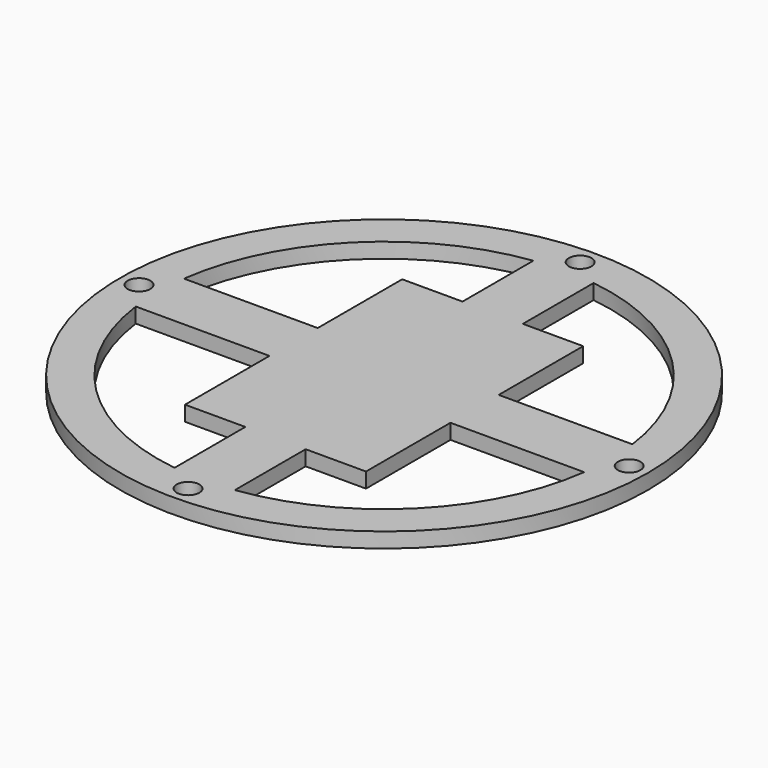
from build123d import *

# Parameters (mm, degrees)
F0_R     = 35
F0_R_2   = 1.5
F0_W     = 19.983293198
F0_H     = 32
F1_DEPTH = 2


# Not quite as in the source:
# - a feature names something its author has since deleted; it is built from what else it names


with BuildPart() as f1:
    # F0 (on Top) → F1 (new body)
    with BuildSketch(Plane.XY):
        Circle(F0_R)
        with Locations((0, -32.5)):
            Circle(F0_R_2, mode=Mode.SUBTRACT)
        with Locations((-32.5, 0)):
            Circle(F0_R_2, mode=Mode.SUBTRACT)
        with BuildLine():
            ThreePointArc((29.7321374946, 4), (29.9329594664, 2.0044793789), (30, 0))
            ThreePointArc((30, 0), (29.9329594664, -2.0044793789), (29.7321374946, -4))
            ThreePointArc((29.7321374946, -4), (21.2132034356, -21.2132034356), (4, -29.7321374946))
            ThreePointArc((4, -29.7321374946), (0, -30), (-4, -29.7321374946))
            ThreePointArc((-4, -29.7321374946), (-21.2132034356, -21.2132034356), (-29.7321374946, -4))
            ThreePointArc((-29.7321374946, -4), (-30, 0), (-29.7321374946, 4))
            ThreePointArc((-29.7321374946, 4), (-21.2132034356, 21.2132034356), (-4, 29.7321374946))
            ThreePointArc((-4, 29.7321374946), (0, 30), (4, 29.7321374946))
            ThreePointArc((4, 29.7321374946), (21.2132034356, 21.2132034356), (29.7321374946, 4))
        make_face(mode=Mode.SUBTRACT)
        with Locations((32.5, 0)):
            Circle(F0_R_2, mode=Mode.SUBTRACT)
        with Locations((0, 32.5)):
            Circle(F0_R_2, mode=Mode.SUBTRACT)
        with BuildLine():
            Line((4, 18), (4, 29.7321374946))
            ThreePointArc((4, 29.7321374946), (0, 30), (-4, 29.7321374946))
            Line((-4, 29.7321374946), (-4, 18))
            Line((-4, 18), (4, 18))
        make_face()
        with BuildLine():
            Line((-12, 4), (-29.7321374946, 4))
            ThreePointArc((-29.7321374946, 4), (-30, 0), (-29.7321374946, -4))
            Line((-29.7321374946, -4), (-12, -4))
            Line((-12, -4), (-12, 4))
        make_face()
        with BuildLine():
            ThreePointArc((-4, -29.7321374946), (0, -30), (4, -29.7321374946))
            Line((4, -29.7321374946), (4, -18))
            Line((4, -18), (-4, -18))
            Line((-4, -18), (-4, -29.7321374946))
        make_face()
        Polygon((12, -4), (12, 4), (12, 12.1005004627), (12, 18), (4, 18), (-4, 18), (-12, 18), (-12, 4), (-12, -4), (-12, -18), (-4, -18), (4, -18), (12, -18), (12, -5.151443038), align=None)
        with Locations((0.1530251862, 0.242334145)):
            Rectangle(F0_W, F0_H, mode=Mode.SUBTRACT)
        with Locations((0.1530251862, 0.242334145)):
            Rectangle(F0_W, F0_H)
        with BuildLine():
            ThreePointArc((29.7321374946, -4), (29.9329594664, -2.0044793789), (30, 0))
            ThreePointArc((30, 0), (29.9329594664, 2.0044793789), (29.7321374946, 4))
            Line((29.7321374946, 4), (12, 4))
            Line((12, 4), (12, -4))
            Line((12, -4), (29.7321374946, -4))
        make_face()
    extrude(amount=F1_DEPTH)


solid = f1.part
